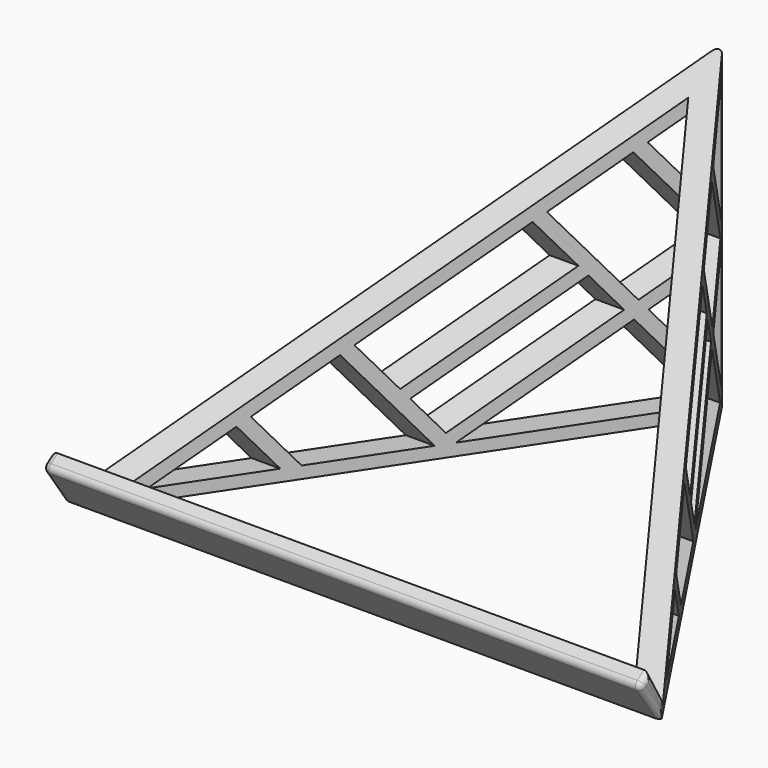
from build123d import *

# Parameters (mm, degrees)
F3_DEPTH      = 131.9225803607
F4_DEPTH      = 125.001
F4_DEPTH_BACK = 125.001
F5_DEPTH      = 125
F5_DEPTH_BACK = 125
F6_DEPTH      = 131.9235803607
F7_T1_DEPTH   = 245
F7_T3_DEPTH   = 150.7630773794
F7_T5_DEPTH   = 13.7314992305
F7_T7_DEPTH   = 28.125
F7_T9_DEPTH   = 28.759876308
F7_T11_DEPTH  = 10.4997732705
F7_S15_W      = 2.5
F7_S15_H      = 2.5
F7_T16_DEPTH  = 2.5
F7_S21_W      = 2.5
F7_S21_H      = 2.5
F7_T22_DEPTH  = 2.5


# Not quite as in the source:
# - a fillet or chamfer that OpenCascade refuses, or shapes differently, is made with other operations: its cross-section is extruded or revolved along the edge and cut away or added
# - a feature names something its author has since deleted; it is built from what else it names


with BuildPart() as f3:
    # F2 (on Top) → F3 (new body, through all)
    with BuildSketch(Plane.XY):
        Polygon((0, 188.4049701865), (-125, 0), (125, 0), align=None)
        Polygon((106.3645843666, 10), (-106.3645843666, 10), (0, 170.3169307719), align=None, mode=Mode.SUBTRACT)
    extrude(amount=F3_DEPTH)

    # F1 (on Right) → F4 (cut, two sides)
    with BuildSketch(Plane.YZ) as f4_sk:
        Polygon((53.8201586062, 5), (41.330982217, 22.8363923661), (15.8579740118, 5), align=None)
        Polygon((97.8862161444, 5), (70.8997506436, 43.540666914), (45.4267424384, 25.7042745479), (59.92403155, 5), align=None)
        Polygon((138.9380673151, 63.378159939), (125.8747192944, 82.0345543761), (74.995510865, 46.4085490958), (88.0588588857, 27.7521546586), align=None)
        Polygon((101.1222069064, 9.0957602214), (152.0014153358, 44.7217655018), (141.8059494968, 59.2823997175), (90.9267410675, 23.6563944372), align=None)
        Polygon((179.8148949712, 5), (154.8692975175, 40.6260052804), (103.9900890882, 5), align=None)
        Polygon((183.4049701865, 8.5900752153), (183.4049701865, 60.606898391), (158.965057739, 43.4938874621), align=None)
        Polygon((156.0971755572, 47.5896476836), (180.7665407818, 64.8633231767), (154.6398447404, 102.176112051), (129.9704795158, 84.9024365579), align=None)
        Polygon((183.4049701865, 69.8124894596), (183.4049701865, 122.3176697259), (158.7356049619, 105.0439942328), align=None)
        Polygon((0, 9.9619469809), (0, 0), (4.0957602214, 2.8678821818), align=None)
        Polygon((0, 9.9619469809), (4.0957602214, 2.8678821818), (188.4049701865, 131.9225803607), (0, 131.9225803607), align=None)
    extrude(amount=-F4_DEPTH, mode=Mode.SUBTRACT)
    extrude(f4_sk.sketch, amount=F4_DEPTH_BACK, mode=Mode.SUBTRACT)

    # F1 (on Right) → F5 (join, two sides)
    with BuildSketch(Plane.YZ) as f5_sk:
        Polygon((-11.471528727, 16.3830408858), (0, 0), (0, 9.9619469809), (-5.942438154, 20.2545517845), align=None)
        Polygon((0, 9.9619469809), (0, 0), (4.0957602214, 2.8678821818), align=None)
    extrude(amount=F5_DEPTH)
    extrude(f5_sk.sketch, amount=-F5_DEPTH_BACK)

    # F2 (on Top) → F6 (cut, through all)
    with BuildSketch(Plane.XY):
        Polygon((-125, 188.4049701865), (-125, 0), (0, 188.4049701865), align=None)
        Polygon((0, 188.4049701865), (125, 0), (125, 188.4049701865), align=None)
    extrude(amount=F6_DEPTH, mode=Mode.SUBTRACT)

    # F7: fillet of radius 2.5 on 10 edges, made by hand

    # F7_s2 → F7_t1 (cut)
    with BuildSketch(Plane.YZ.offset(-122.5)):
        with BuildLine():
            ThreePointArc((-10.0375876361, 14.3351607751), (-10.451726908, 16.2032223101), (-9.4236486163, 17.8169819767))
            Line((-9.4236486163, 17.8169819767), (-11.471528727, 16.3830408858))
            Line((-11.471528727, 16.3830408858), (-10.0375876361, 14.3351607751))
        make_face()
    extrude(amount=F7_T1_DEPTH, mode=Mode.SUBTRACT)

    # F7_s4 → F7_t3 (cut)
    with BuildSketch(Plane.XY.offset(-9.4202485093)):
        with BuildLine():
            ThreePointArc((-2.0831994653, 185.2650891212), (0, 186.3829603328), (2.0831994653, 185.2650891212))
            Line((2.0831994653, 185.2650891212), (0, 188.4049701865))
            Line((0, 188.4049701865), (-2.0831994653, 185.2650891212))
        make_face()
    extrude(amount=F7_T3_DEPTH, mode=Mode.SUBTRACT)

    # F7_s6 → F7_t5 (cut)
    with BuildSketch(Plane.XY.offset(-1.8847761248)):
        with BuildLine():
            ThreePointArc((-124.5831994653, 0.6282183385), (-124.893532814, -0.0321066896), (-125, -0.7539104499))
            Line((-125, -0.7539104499), (-125, 0))
            Line((-125, 0), (-124.5831994653, 0.6282183385))
        make_face()
        with BuildLine():
            ThreePointArc((124.5831994653, 0.6282183385), (124.893532814, -0.0321066896), (125, -0.7539104499))
            Line((125, -0.7539104499), (125, 0))
            Line((125, 0), (124.5831994653, 0.6282183385))
        make_face()
    extrude(amount=F7_T5_DEPTH, mode=Mode.SUBTRACT)

    # F7_s8 → F7_t7 (cut)
    with BuildSketch(Plane(origin=(0, -10.0375876361, 14.3351607751), x_dir=(1, 0, 0), z_dir=(0, 0.5735764364, -0.8191520443))):
        with BuildLine():
            ThreePointArc((122.5, 0), (124.267766953, -0.732233047), (125, -2.5))
            Line((125, -2.5), (125, 0))
            Line((125, 0), (122.5, 0))
        make_face()
        with BuildLine():
            ThreePointArc((-122.5, 0), (-124.267766953, -0.732233047), (-125, -2.5))
            Line((-125, -2.5), (-125, 0))
            Line((-125, 0), (-122.5, 0))
        make_face()
    extrude(amount=F7_T7_DEPTH, mode=Mode.SUBTRACT)

    # F7_s10 → F7_t9 (cut)
    with BuildSketch(Plane(origin=(0, 0.9988504217, -1.7300596795), x_dir=(1, 0, 0), z_dir=(0, -0.5, 0.8660254038))):
        with BuildLine():
            ThreePointArc((-122.5, 4.9809734905), (-124.267766953, 4.2487404434), (-125, 2.4809734905))
            Line((-125, 2.4809734905), (-125, 4.9809734905))
            Line((-125, 4.9809734905), (-122.5, 4.9809734905))
        make_face()
        with BuildLine():
            ThreePointArc((122.5, 4.9809734905), (124.267766953, 4.2487404434), (125, 2.4809734905))
            Line((125, 2.4809734905), (125, 4.9809734905))
            Line((125, 4.9809734905), (122.5, 4.9809734905))
        make_face()
    extrude(amount=F7_T9_DEPTH, mode=Mode.SUBTRACT)

    # F7_s12 → F7_t11 (cut)
    with BuildSketch(Plane(origin=(0, 10.6487908498, 7.4563636259), x_dir=(1, 0, 0), z_dir=(0, -0.8191520443, -0.5735764364))):
        with BuildLine():
            ThreePointArc((-125, 17.5), (-124.267766953, 19.267766953), (-122.5, 20))
            Line((-122.5, 20), (-125, 20))
            Line((-125, 20), (-125, 17.5))
        make_face()
        with BuildLine():
            ThreePointArc((125, 17.5), (124.267766953, 19.267766953), (122.5, 20))
            Line((122.5, 20), (125, 20))
            Line((125, 20), (125, 17.5))
        make_face()
    extrude(amount=F7_T11_DEPTH, mode=Mode.SUBTRACT)


with BuildPart() as f7_tool14:
    # F7_s15 → F7_t16 (new body)
    with BuildSketch(Plane(origin=(0, 2.0478801107, 1.4339410909), x_dir=(1, 0, 0), z_dir=(0, -0.8191520443, -0.5735764364))):
        with Locations((-123.75, 18.75)):
            Rectangle(F7_S15_W, F7_S15_H)
    extrude(amount=F7_T16_DEPTH)

    # F7_s17 → F7_t18 (revolve, cut)
    with BuildSketch(Plane(origin=(-122.5, -7.9897075254, 15.7691018659), x_dir=(0.7071067812, 0.4055797877, -0.5792279653), z_dir=(-0.7071067812, 0.4055797877, -0.5792279653))):
        with BuildLine():
            ThreePointArc((0, -2.5), (2.5, 0), (0, 2.5))
            Line((0, 2.5), (0, -2.5))
        make_face()
    revolve(axis=Axis((-122.5, -7.9897075254, 15.7691018659), (0, -0.8191520443, -0.5735764364)), mode=Mode.SUBTRACT)


with BuildPart() as f3_1:
    add(f3.part)

    # F7_t13: cut F7_tool14
    add(f7_tool14.part, mode=Mode.SUBTRACT)


with BuildPart() as f7_tool20:
    # F7_s21 → F7_t22 (new body)
    with BuildSketch(Plane(origin=(0, 2.0478801107, 1.4339410909), x_dir=(1, 0, 0), z_dir=(0, -0.8191520443, -0.5735764364))):
        with Locations((123.75, 18.75)):
            Rectangle(F7_S21_W, F7_S21_H)
    extrude(amount=F7_T22_DEPTH)

    # F7_s23 → F7_t24 (revolve, cut)
    with BuildSketch(Plane(origin=(122.5, -7.9897075254, 15.7691018659), x_dir=(-0.7071067812, 0.4055797877, -0.5792279653), z_dir=(-0.7071067812, -0.4055797877, 0.5792279653))):
        with BuildLine():
            ThreePointArc((0, -2.5), (2.5, 0), (0, 2.5))
            Line((0, 2.5), (0, -2.5))
        make_face()
    revolve(axis=Axis((122.5, -7.9897075254, 15.7691018659), (0, -0.8191520443, -0.5735764364)), mode=Mode.SUBTRACT)


with BuildPart() as f3_2:
    add(f3_1.part)

    # F7_t19: cut F7_tool20
    add(f7_tool20.part, mode=Mode.SUBTRACT)


solid = f3_2.part
